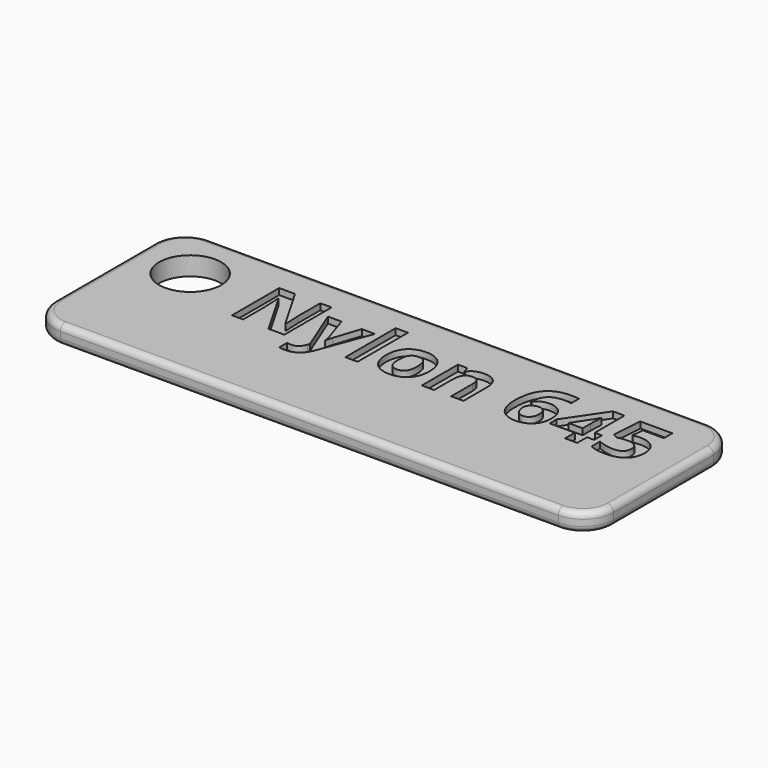
from build123d import *

# Parameters (mm, degrees)
F0_W         = 90
F0_H         = 30
F1_DEPTH     = 3
F2_R         = 1
F3_T3_ANGLE  = 90
F3_T6_ANGLE  = 90
F3_T9_ANGLE  = 90
F3_T12_ANGLE = 90
F3_T15_ANGLE = 90
F3_T18_ANGLE = 90
F3_T21_ANGLE = 90
F3_T24_ANGLE = 90
F3_T27_DEPTH = 3
F3_T30_DEPTH = 3
F3_T33_DEPTH = 3
F3_T36_DEPTH = 3
F4_R         = 5
F5_DEPTH     = 3
F6_TEXT_SIZE = 13.3181990163
F7_DEPTH     = 1


# Not quite as in the source:
# - a fillet or chamfer that OpenCascade refuses, or shapes differently, is made with other operations: its cross-section is extruded or revolved along the edge and cut away or added
# - Text() gives the source's letters only with a copy of the font that has no kerning and outlines rounded to 1/6400 em; it was checked with that copy


with BuildPart() as f1:
    # F0 (on Top) → F1 (new body)
    with BuildSketch(Plane.XY):
        Rectangle(F0_W, F0_H)
    extrude(amount=F1_DEPTH)

    # F2
    f2_edges = [f1.edges().sort_by_distance(p)[0] for p in [
        (0, 15, 3),
        (-45, 0, 3),
        (0, -15, 3),
        (45, 0, 3),
        (0, 15, 0),
        (-45, 0, 0),
        (0, -15, 0),
        (45, 0, 0),
    ]]
    fillet(f2_edges, radius=F2_R)

    # F3: fillet of radius 5 on 4 edges, made by hand


with BuildPart() as f3_tool1:
    # F3_s2 → F3_t3 (revolve)
    with BuildSketch(Plane.YZ.offset(-39.9990343146)):
        with BuildLine():
            ThreePointArc((-14.0004, 0), (-14.7075067812, 0.2928932188), (-15.0004, 1))
            Line((-15.0004, 1), (-15.0004, 0))
            Line((-15.0004, 0), (-14.0004, 0))
        make_face()
    revolve(axis=Axis((-39.9990343146, -9.9990343146, 0), (0, 0, -1)), revolution_arc=F3_T3_ANGLE)


with BuildPart() as f3_tool4:
    # F3_s5 → F3_t6 (revolve)
    with BuildSketch(Plane.XZ.offset(9.9990343146)):
        with BuildLine():
            ThreePointArc((-44.0004, 3), (-44.7075067812, 2.7071067812), (-45.0004, 2))
            Line((-45.0004, 2), (-45.0004, 3))
            Line((-45.0004, 3), (-44.0004, 3))
        make_face()
    revolve(axis=Axis((-39.9990343146, -9.9990343146, 3), (0, 0, 1)), revolution_arc=F3_T6_ANGLE)


with BuildPart() as f3_tool7:
    # F3_s8 → F3_t9 (revolve)
    with BuildSketch(Plane.XZ.offset(-9.9990343146)):
        with BuildLine():
            ThreePointArc((-44.0004, 0), (-44.7075067812, 0.2928932188), (-45.0004, 1))
            Line((-45.0004, 1), (-45.0004, 0))
            Line((-45.0004, 0), (-44.0004, 0))
        make_face()
    revolve(axis=Axis((-39.9990343146, 9.9990343146, 0), (0, 0, -1)), revolution_arc=F3_T9_ANGLE)


with BuildPart() as f3_tool10:
    # F3_s11 → F3_t12 (revolve)
    with BuildSketch(Plane.YZ.offset(-39.9990343146)):
        with BuildLine():
            ThreePointArc((14.0004, 3), (14.7075067812, 2.7071067812), (15.0004, 2))
            Line((15.0004, 2), (15.0004, 3))
            Line((15.0004, 3), (14.0004, 3))
        make_face()
    revolve(axis=Axis((-39.9990343146, 9.9990343146, 3), (0, 0, 1)), revolution_arc=F3_T12_ANGLE)


with BuildPart() as f3_tool13:
    # F3_s14 → F3_t15 (revolve)
    with BuildSketch(Plane.YZ.offset(39.9990343146)):
        with BuildLine():
            ThreePointArc((14.0004, 0), (14.7075067812, 0.2928932188), (15.0004, 1))
            Line((15.0004, 1), (15.0004, 0))
            Line((15.0004, 0), (14.0004, 0))
        make_face()
    revolve(axis=Axis((39.9990343146, 9.9990343146, 0), (0, 0, -1)), revolution_arc=F3_T15_ANGLE)


with BuildPart() as f3_tool16:
    # F3_s17 → F3_t18 (revolve)
    with BuildSketch(Plane.XZ.offset(-9.9990343146)):
        with BuildLine():
            ThreePointArc((44.0004, 3), (44.7075067812, 2.7071067812), (45.0004, 2))
            Line((45.0004, 2), (45.0004, 3))
            Line((45.0004, 3), (44.0004, 3))
        make_face()
    revolve(axis=Axis((39.9990343146, 9.9990343146, 3), (0, 0, 1)), revolution_arc=F3_T18_ANGLE)


with BuildPart() as f3_tool19:
    # F3_s20 → F3_t21 (revolve)
    with BuildSketch(Plane.XZ.offset(9.9990343146)):
        with BuildLine():
            ThreePointArc((44.0004, 0), (44.7075067812, 0.2928932188), (45.0004, 1))
            Line((45.0004, 1), (45.0004, 0))
            Line((45.0004, 0), (44.0004, 0))
        make_face()
    revolve(axis=Axis((39.9990343146, -9.9990343146, 0), (0, 0, -1)), revolution_arc=F3_T21_ANGLE)


with BuildPart() as f3_tool22:
    # F3_s23 → F3_t24 (revolve)
    with BuildSketch(Plane.YZ.offset(39.9990343146)):
        with BuildLine():
            ThreePointArc((-14.0004, 3), (-14.7075067812, 2.7071067812), (-15.0004, 2))
            Line((-15.0004, 2), (-15.0004, 3))
            Line((-15.0004, 3), (-14.0004, 3))
        make_face()
    revolve(axis=Axis((39.9990343146, -9.9990343146, 3), (0, 0, 1)), revolution_arc=F3_T24_ANGLE)


with BuildPart() as f3_tool25:
    # F3_s26 → F3_t27 (new body)
    with BuildSketch(Plane.XY):
        with BuildLine():
            ThreePointArc((45.0004, -9.9990343146), (43.5355339059, -13.5355339059), (39.9990343146, -15.0004))
            Line((39.9990343146, -15.0004), (39.9990343146, -15.5005365685))
            ThreePointArc((39.9990343146, -15.5005365685), (42.4995171573, -15.5001365685), (45, -15.5001365685))
            Line((45, -15.5001365685), (45.5001365685, -15))
            ThreePointArc((45.5001365685, -15), (45.5001365685, -12.4995171573), (45.5005365685, -9.9990343146))
            Line((45.5005365685, -9.9990343146), (45.0004, -9.9990343146))
        make_face()
    extrude(amount=F3_T27_DEPTH)


with BuildPart() as f3_tool28:
    # F3_s29 → F3_t30 (new body)
    with BuildSketch(Plane.XY):
        with BuildLine():
            ThreePointArc((39.9990343146, 15.0004), (43.5355339059, 13.5355339059), (45.0004, 9.9990343146))
            Line((45.0004, 9.9990343146), (45.5005365685, 9.9990343146))
            ThreePointArc((45.5005365685, 9.9990343146), (45.5001365685, 12.4995171573), (45.5001365685, 15))
            Line((45.5001365685, 15), (45, 15.5001365685))
            ThreePointArc((45, 15.5001365685), (42.4995171573, 15.5001365685), (39.9990343146, 15.5005365685))
            Line((39.9990343146, 15.5005365685), (39.9990343146, 15.0004))
        make_face()
    extrude(amount=F3_T30_DEPTH)


with BuildPart() as f3_tool31:
    # F3_s32 → F3_t33 (new body)
    with BuildSketch(Plane.XY):
        with BuildLine():
            ThreePointArc((-39.9990343146, 15.0004), (-43.5355339059, 13.5355339059), (-45.0004, 9.9990343146))
            Line((-45.0004, 9.9990343146), (-45.5005365685, 9.9990343146))
            ThreePointArc((-45.5005365685, 9.9990343146), (-45.5001365685, 12.4995171573), (-45.5001365685, 15))
            Line((-45.5001365685, 15), (-45, 15.5001365685))
            ThreePointArc((-45, 15.5001365685), (-42.4995171573, 15.5001365685), (-39.9990343146, 15.5005365685))
            Line((-39.9990343146, 15.5005365685), (-39.9990343146, 15.0004))
        make_face()
    extrude(amount=F3_T33_DEPTH)


with BuildPart() as f3_tool34:
    # F3_s35 → F3_t36 (new body)
    with BuildSketch(Plane.XY):
        with BuildLine():
            ThreePointArc((-45.0004, -9.9990343146), (-43.5355339059, -13.5355339059), (-39.9990343146, -15.0004))
            Line((-39.9990343146, -15.0004), (-39.9990343146, -15.5005365685))
            ThreePointArc((-39.9990343146, -15.5005365685), (-42.4995171573, -15.5001365685), (-45, -15.5001365685))
            Line((-45, -15.5001365685), (-45.5001365685, -15))
            ThreePointArc((-45.5001365685, -15), (-45.5001365685, -12.4995171573), (-45.5005365685, -9.9990343146))
            Line((-45.5005365685, -9.9990343146), (-45.0004, -9.9990343146))
        make_face()
    extrude(amount=F3_T36_DEPTH)


with BuildPart() as f1_1:
    add(f1.part)

    # F3_t37: cut F3_tool1, F3_tool4, F3_tool7, F3_tool10, F3_tool13, F3_tool16, F3_tool19, F3_tool22, F3_tool25, F3_tool28, F3_tool31, F3_tool34
    add([f3_tool1.part, f3_tool4.part, f3_tool7.part, f3_tool10.part, f3_tool13.part, f3_tool16.part, f3_tool19.part, f3_tool22.part, f3_tool25.part, f3_tool28.part, f3_tool31.part, f3_tool34.part], mode=Mode.SUBTRACT)

    # F4 (on face) → F5 (cut)
    with BuildSketch(Plane.XY.offset(3)):
        with Locations((-36, 6)):
            Circle(F4_R)
    extrude(amount=-F5_DEPTH, mode=Mode.SUBTRACT)

    # F6 (on face) → F7 (cut)
    with BuildSketch(Plane.XY.offset(3)):
        with Locations((-26, 0.4108967083)):
            Text('Nylon 645', F6_TEXT_SIZE, font='Open Sans', font_style=FontStyle.BOLD, text_align=(TextAlign.LEFT, TextAlign.BOTTOM))
    extrude(amount=-F7_DEPTH, mode=Mode.SUBTRACT)


solid = f1_1.part
